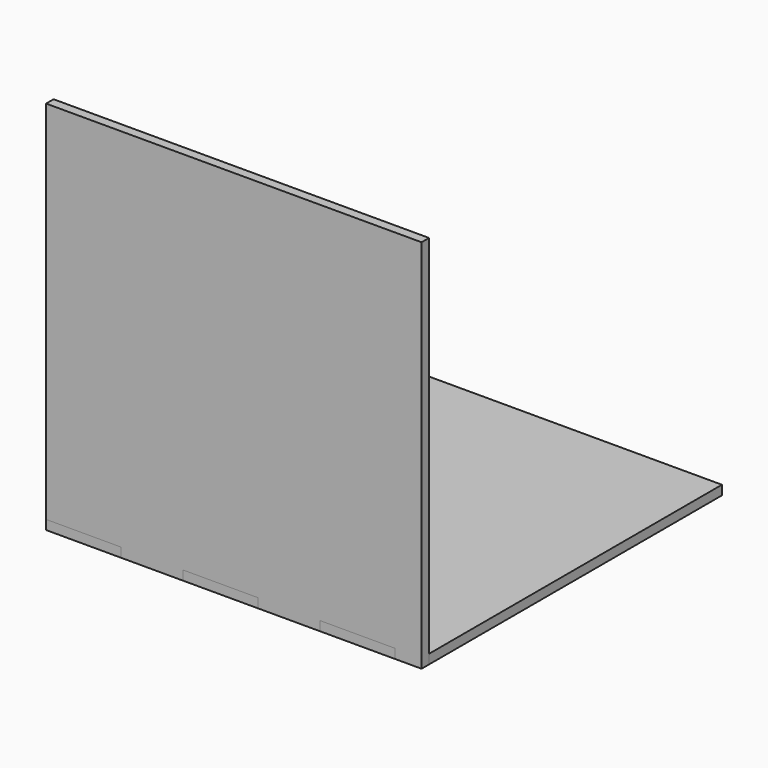
from build123d import *

# Parameters (mm, degrees)
F0_W     = 127
F0_H     = 127
F1_DEPTH = 3.175
F2_W     = 127
F2_H     = 3.175
F3_DEPTH = 127
F4_W     = 25.3358542953
F4_H     = 3.175
F4_W_2   = 25.4
F5_DEPTH = 25.4


with BuildPart() as f1:
    # F0 (on Top) → F1 (new body)
    with BuildSketch(Plane.XY):
        Rectangle(F0_W, F0_H)
    extrude(amount=F1_DEPTH)


with BuildPart() as f3:
    # F2 (on Top) → F3 (new body)
    with BuildSketch(Plane.XY):
        with Locations((0, -61.9125)):
            Rectangle(F2_W, F2_H)
    extrude(amount=F3_DEPTH)

    # F4 (on face) → F5 (cut)
    with BuildSketch(Plane.XZ.offset(63.5)):
        with Locations((-50.8320728524, 1.5875)):
            Rectangle(F4_W, F4_H)
        with Locations((-4.5091457047, 1.5875)):
            Rectangle(F4_W_2, F4_H)
        with Locations((41.8458542953, 1.5875)):
            Rectangle(F4_W_2, F4_H)
    extrude(amount=-F5_DEPTH, mode=Mode.SUBTRACT)


solid = Compound([f1.part, f3.part])
